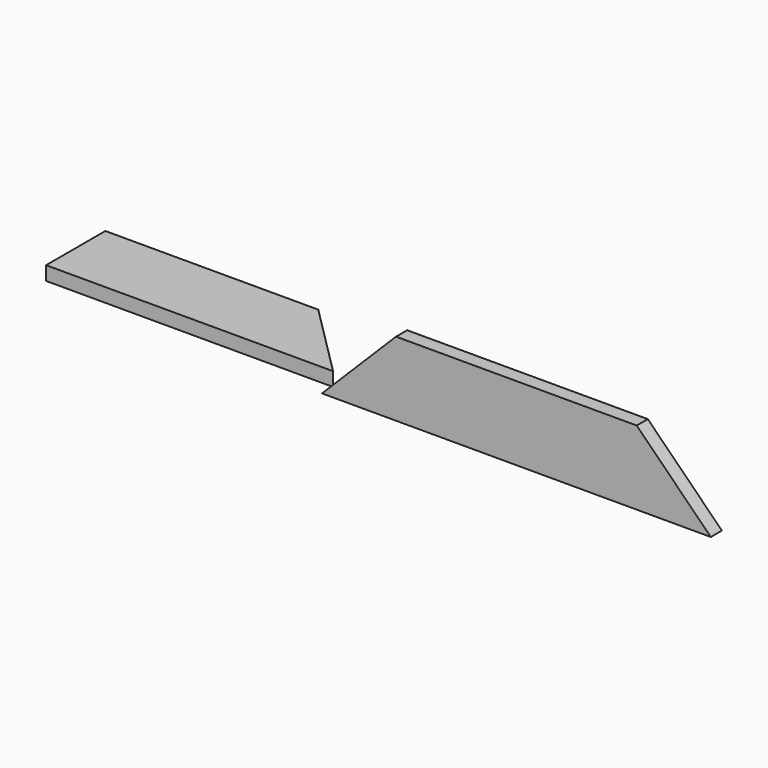
from build123d import *

# Parameters (mm, degrees)
F0_W     = 266.7
F0_H     = 50.8
F1_DEPTH = 9.525
F2_SIZE  = 50.79999
F3_W     = 196.85
F3_H     = 50.8
F4_DEPTH = 9.525
F5_SIZE  = 50.79999


# Not quite as in the source:
# - a fillet or chamfer is up to 0.001 mm smaller than in the source, because OpenCascade refuses the exact size


with BuildPart() as f1:
    # F0 (on Front) → F1 (new body)
    with BuildSketch(Plane.XZ):
        with Locations((133.35, 25.4)):
            Rectangle(F0_W, F0_H)
    extrude(amount=F1_DEPTH)

    # F2 (size 50.8 in the source; OpenCascade refuses exactly that, so slightly less here)
    f2_edges = [f1.edges().sort_by_distance(p)[0] for p in [
        (266.7, -4.7625, 50.8),
        (0, -4.7625, 50.8),
    ]]
    chamfer(f2_edges, length=F2_SIZE)


with BuildPart() as f4:
    # F3 (on Top) → F4 (new body)
    with BuildSketch(Plane.XY):
        with Locations((-98.425, 25.4)):
            Rectangle(F3_W, F3_H)
    extrude(amount=F4_DEPTH)

    # F5 (size 50.8 in the source; OpenCascade refuses exactly that, so slightly less here)
    f5_edges = [f4.edges().sort_by_distance(p)[0] for p in [
        (0, 50.8, 4.7625),
    ]]
    chamfer(f5_edges, length=F5_SIZE)


solid = Compound([f1.part, f4.part])
